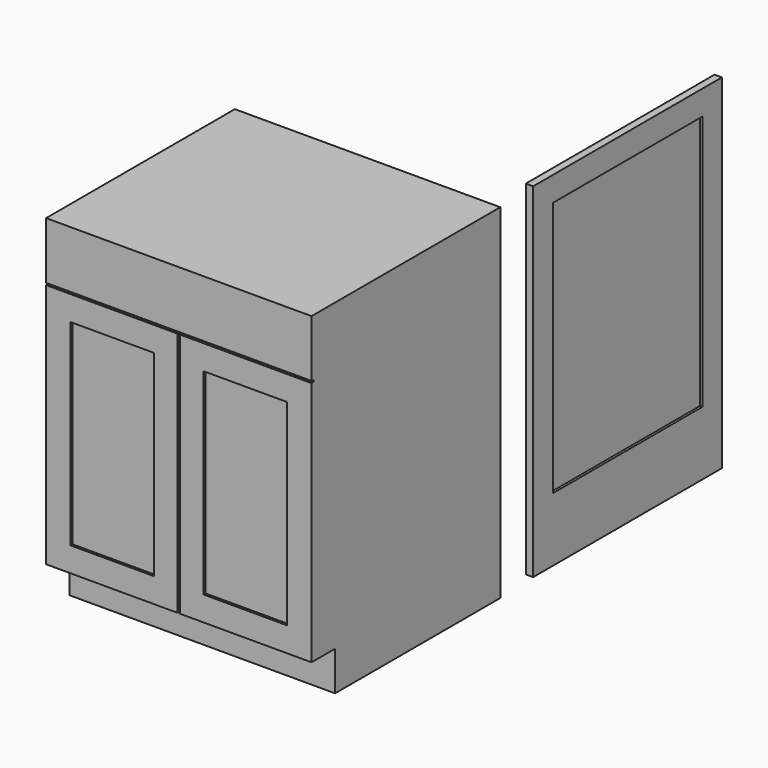
from build123d import *

# Parameters (mm, degrees)
F0_W     = 3.175
F0_H     = 635
F0_W_2   = 339.725
F0_W_3   = 215.9
F0_H_2   = 508
F0_W_4   = 342.9
F0_H_3   = 147.32
F1_DEPTH = 609.6
F2_DEPTH = 6.35
F3_DEPTH = 76.2
F4_W     = 609.6
F4_H     = 889
F4_W_2   = 482.6
F4_H_2   = 660.4
F5_DEPTH = 19.05
F6_DEPTH = 12.7


with BuildPart() as f1:
    # F0 (on Front) → F1 (new body)
    with BuildSketch(Plane.XZ):
        Polygon((227.9072425127, -101.6), (227.9072425127, 0), (224.7322425127, 0), (-114.9927574873, 0), (-114.9927574873, -101.6), align=None)
        with Locations((226.3197425127, 317.5)):
            Rectangle(F0_W, F0_H)
        Polygon((231.0822425127, 0), (227.9072425127, 0), (227.9072425127, -101.6), (570.8072425127, -101.6), (570.8072425127, 0), align=None)
        with Locations((229.4947425127, 317.5)):
            Rectangle(F0_W, F0_H)
        with Locations((54.8697425127, 317.5)):
            Rectangle(F0_W_2, F0_H)
        with Locations((56.4572425127, 317.5)):
            Rectangle(F0_W_3, F0_H_2, mode=Mode.SUBTRACT)
        Polygon((224.7322425127, 635), (227.9072425127, 635), (227.9072425127, 640.08), (-114.9927574873, 640.08), (-114.9927574873, 635), align=None)
        Polygon((227.9072425127, 640.08), (227.9072425127, 635), (231.0822425127, 635), (570.8072425127, 635), (570.8072425127, 640.08), align=None)
        with Locations((400.9447425127, 317.5)):
            Rectangle(F0_W_2, F0_H)
        with Locations((399.3572425127, 317.5)):
            Rectangle(F0_W_3, F0_H_2, mode=Mode.SUBTRACT)
        with Locations((56.4572425127, 713.74)):
            Rectangle(F0_W_4, F0_H_3)
        with Locations((399.3572425127, 713.74)):
            Rectangle(F0_W_4, F0_H_3)
        with Locations((56.4572425127, 317.5)):
            Rectangle(F0_W_3, F0_H_2)
        with Locations((399.3572425127, 317.5)):
            Rectangle(F0_W_3, F0_H_2)
    extrude(amount=-F1_DEPTH)

    # F0 (on Front) → F2 (cut)
    with BuildSketch(Plane.XZ):
        with Locations((226.3197425127, 317.5)):
            Rectangle(F0_W, F0_H)
        with Locations((229.4947425127, 317.5)):
            Rectangle(F0_W, F0_H)
        Polygon((224.7322425127, 635), (227.9072425127, 635), (227.9072425127, 640.08), (-114.9927574873, 640.08), (-114.9927574873, 635), align=None)
        Polygon((227.9072425127, 640.08), (227.9072425127, 635), (231.0822425127, 635), (570.8072425127, 635), (570.8072425127, 640.08), align=None)
        with Locations((56.4572425127, 317.5)):
            Rectangle(F0_W_3, F0_H_2)
        with Locations((399.3572425127, 317.5)):
            Rectangle(F0_W_3, F0_H_2)
    extrude(amount=-F2_DEPTH, mode=Mode.SUBTRACT)

    # F0 (on Front) → F3 (cut)
    with BuildSketch(Plane.XZ):
        Polygon((227.9072425127, -101.6), (227.9072425127, 0), (224.7322425127, 0), (-114.9927574873, 0), (-114.9927574873, -101.6), align=None)
        Polygon((231.0822425127, 0), (227.9072425127, 0), (227.9072425127, -101.6), (570.8072425127, -101.6), (570.8072425127, 0), align=None)
    extrude(amount=-F3_DEPTH, mode=Mode.SUBTRACT)


with BuildPart() as f5:
    # F4 (on face) → F5 (new body)
    with BuildSketch(Plane.YZ.offset(570.8072425127)):
        with Locations((996.8526720047, 363.0936748981)):
            Rectangle(F4_W, F4_H)
        with Locations((996.8526720047, 413.8936748981)):
            Rectangle(F4_W_2, F4_H_2, mode=Mode.SUBTRACT)
    extrude(amount=F5_DEPTH)

    # F4 (on face) → F6 (join)
    with BuildSketch(Plane.YZ.offset(570.8072425127)):
        with Locations((996.8526720047, 413.8936748981)):
            Rectangle(F4_W_2, F4_H_2)
    extrude(amount=F6_DEPTH)


solid = Compound([f1.part, f5.part])
